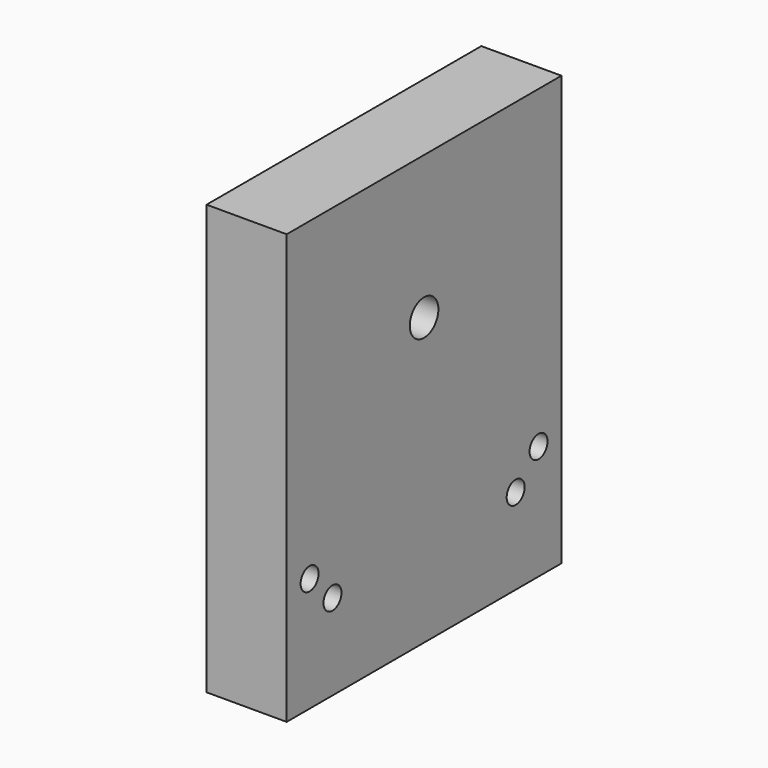
from build123d import *

# Parameters (mm, degrees)
F0_W      = 177.8
F0_H      = 76.2
F1_DEPTH  = 31.75
F2_W      = 19.05
F2_H      = 76.2
F3_DEPTH  = 63.5
F4_W      = 107.95
F4_H      = 38.1
F5_DEPTH  = 31.751
F6_W      = 107.95
F6_H      = 19.05
F7_DEPTH  = 12.7
F8_W      = 76.2
F8_H      = 31.75
F9_DEPTH  = 50.8
F11_D     = 6.5278
F11_DEPTH = 12.7
F11_TIP   = 1.9611489744
F14_D     = 7.9375
F15_W     = 19.05
F15_H     = 19.05
F15_R     = 3.2639
F12_W     = 19.05
F12_H     = 19.05
F12_R     = 3.2639
F16_DEPTH = 107.95
F18_D     = 4.9784
F19_W     = 76.2
F19_H     = 95.25
F19_R     = 2.4892
F19_R_2   = 3.96875
F20_DEPTH = 1.27
F22_D     = 6.9088
F22_DEPTH = 24.3416666667
F22_TIP   = 2.0756129224


with BuildPart() as f1:
    # F0 (on Top) → F1 (new body)
    with BuildSketch(Plane.XY):
        with Locations((88.9, 38.1)):
            Rectangle(F0_W, F0_H)
    extrude(amount=F1_DEPTH)

    # F2 (on face) → F3 (join)
    with BuildSketch(Plane.XY.offset(31.75)):
        with Locations((9.525, 38.1)):
            Rectangle(F2_W, F2_H)
    extrude(amount=F3_DEPTH)

    # F4 (on face) → F5 (cut, through all)
    with BuildSketch(Plane.XY.offset(31.75)):
        with Locations((73.025, 38.1)):
            Rectangle(F4_W, F4_H)
    extrude(amount=-F5_DEPTH, mode=Mode.SUBTRACT)

    # F6 (on face) → F7 (cut)
    with BuildSketch(Plane(origin=(0, 0, 0), x_dir=(1, 0, 0), z_dir=(0, 0, -1))):
        with Locations((73.025, -9.525)):
            Rectangle(F6_W, F6_H)
        with Locations((73.025, -66.675)):
            Rectangle(F6_W, F6_H)
    extrude(amount=-F7_DEPTH, mode=Mode.SUBTRACT)

    # F8 (on face) → F9 (cut)
    with BuildSketch(Plane.YZ.offset(177.8)):
        with Locations((38.1, 15.875)):
            Rectangle(F8_W, F8_H)
    extrude(amount=-F9_DEPTH, mode=Mode.SUBTRACT)

    # F11
    with Locations(Plane.YZ.offset(127)):
        with Locations((66.675, 22.225), (9.525, 22.225)):
            Hole(F11_D / 2, depth=F11_DEPTH)
            with Locations((0, 0, -(F11_DEPTH + F11_TIP / 2))):  # 118° drill point
                Cone(0, F11_D / 2, F11_TIP, mode=Mode.SUBTRACT)

    # F14 (through all)
    with Locations(Plane(origin=(0, 0, 0), x_dir=(0, -1, 0), z_dir=(-1, 0, 0))):
        with Locations((-38.1, 63.5)):
            Hole(F14_D / 2)

    # F15 (on face) + F12 (on face) → F16 (cut)
    with BuildSketch(Plane.YZ.offset(127)):
        with Locations((66.675, 22.225)):
            Rectangle(F15_W, F15_H)
        with Locations((66.675, 22.225)):
            Circle(F15_R, mode=Mode.SUBTRACT)
        with Locations((9.525, 22.225)):
            Rectangle(F15_W, F15_H)
        with Locations((9.525, 22.225)):
            Circle(F15_R, mode=Mode.SUBTRACT)
        with Locations((9.525, 22.225)):
            Circle(F15_R)
    with BuildSketch(Plane.YZ.offset(127)):
        with Locations((66.675, 22.225)):
            Rectangle(F12_W, F12_H)
        with Locations((66.675, 22.225)):
            Circle(F12_R, mode=Mode.SUBTRACT)
        with Locations((66.675, 22.225)):
            Circle(F12_R)
    extrude(amount=-F16_DEPTH, mode=Mode.SUBTRACT)

    # F18 (through all)
    with Locations(Plane.YZ.offset(19.05)):
        with Locations((6.35, 25.4), (12.7, 19.05), (63.5, 19.05), (69.85, 25.4)):
            Hole(F18_D / 2)

    # F19 (on face) → F20 (cut)
    with BuildSketch(Plane(origin=(0, 0, 0), x_dir=(0, -1, 0), z_dir=(-1, 0, 0))):
        with Locations((-38.1, 47.625)):
            Rectangle(F19_W, F19_H)
        with Locations((-63.5, 19.05)):
            Circle(F19_R, mode=Mode.SUBTRACT)
        with Locations((-69.85, 25.4)):
            Circle(F19_R, mode=Mode.SUBTRACT)
        with Locations((-12.7, 19.05)):
            Circle(F19_R, mode=Mode.SUBTRACT)
        with Locations((-6.35, 25.4)):
            Circle(F19_R, mode=Mode.SUBTRACT)
        with Locations((-38.1, 63.5)):
            Circle(F19_R_2, mode=Mode.SUBTRACT)
    extrude(amount=-F20_DEPTH, mode=Mode.SUBTRACT)

    # F22
    with Locations(Plane(origin=(0, 0, 0), x_dir=(1, 0, 0), z_dir=(0, 0, -1))):
        with Locations((10.16, -38.1)):
            Hole(F22_D / 2, depth=F22_DEPTH)
            with Locations((0, 0, -(F22_DEPTH + F22_TIP / 2))):  # 118° drill point
                Cone(0, F22_D / 2, F22_TIP, mode=Mode.SUBTRACT)


solid = f1.part
